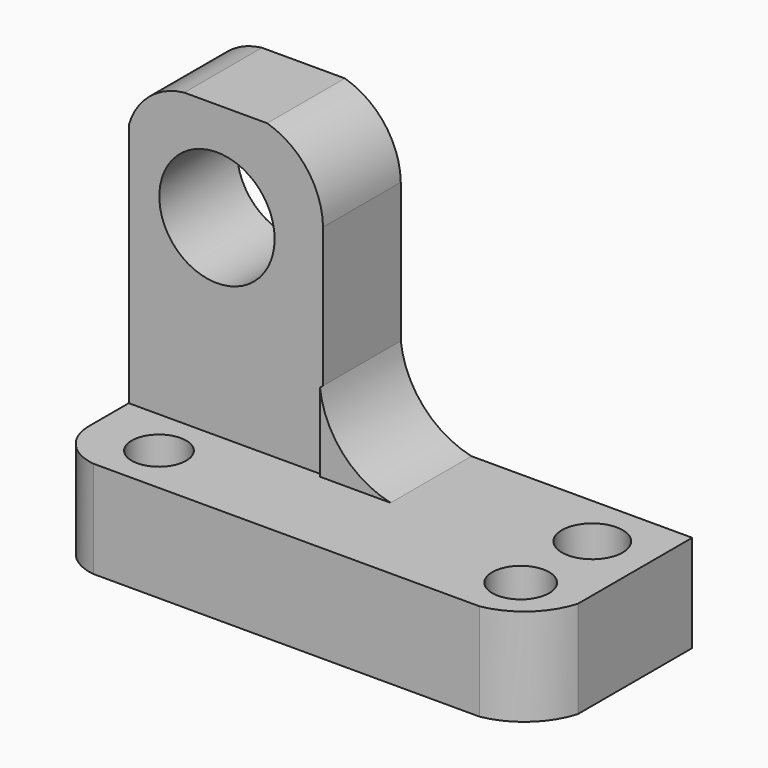
from build123d import *

# Parameters (mm, degrees)
F1_DEPTH  = 25.4
F3_DEPTH  = 25.4
F5_DEPTH  = 12.7
F6_R      = 7.5359717886
F7_DEPTH  = 25.4
F9_DEPTH  = 25.4
F11_DEPTH = 13.208
F12_R     = 3.5651940515
F12_R_2   = 3.719082418
F13_DEPTH = 25.4
F14_R     = 3.972943494
F15_DEPTH = 25.4


# Not quite as in the source:
# - a feature names something its author has since deleted; it is built from what else it names


with BuildPart() as f1:
    # F0 (on Front) → F1 (new body)
    with BuildSketch(Plane.XZ):
        Polygon((-56.0294090864, 50.8), (-56.0294090864, 0), (7.4705909136, 0), (7.4705909136, 12.7), (-30.6294090864, 12.7), (-30.6294090864, 50.8), align=None)
    extrude(amount=F1_DEPTH)

    # F2 (on face) → F3 (cut)
    with BuildSketch(Plane.XZ.offset(25.4)):
        with BuildLine():
            ThreePointArc((-56.0294090864, 44.6911064088), (-53.33876103, 48.8568702153), (-48.7761497498, 50.8))
            Line((-48.7761497498, 50.8), (-56.0294090864, 50.8))
            Line((-56.0294090864, 50.8), (-56.0294090864, 44.6911064088))
        make_face()
        with BuildLine():
            Line((-30.6294090864, 50.8), (-37.9370041192, 50.8))
            ThreePointArc((-37.9370041192, 50.8), (-32.7129588614, 47.2060747706), (-30.6294090864, 41.2172712386))
            Line((-30.6294090864, 41.2172712386), (-30.6294090864, 50.8))
        make_face()
    extrude(amount=-F3_DEPTH, mode=Mode.SUBTRACT)

    # F4 (on face) → F5 (cut)
    with BuildSketch(Plane.XZ.offset(25.4)):
        with BuildLine():
            Line((-56.0294090864, 12.7), (-30.6294090864, 12.7))
            Line((-30.6294090864, 12.7), (-30.6294090864, 41.2172712386))
            ThreePointArc((-30.6294090864, 41.2172712386), (-32.7129588614, 47.2060747706), (-37.9370041192, 50.8))
            Line((-37.9370041192, 50.8), (-48.7761497498, 50.8))
            ThreePointArc((-48.7761497498, 50.8), (-53.33876103, 48.8568702153), (-56.0294090864, 44.6911064088))
            Line((-56.0294090864, 44.6911064088), (-56.0294090864, 12.7))
        make_face()
    extrude(amount=-F5_DEPTH, mode=Mode.SUBTRACT)

    # F6 (on face) → F7 (cut)
    with BuildSketch(Plane.XZ.offset(12.7)):
        with Locations((-44.4975420833, 37.7943851054)):
            Circle(F6_R)
    extrude(amount=-F7_DEPTH, mode=Mode.SUBTRACT)

    # F8 (on face) → F9 (cut)
    with BuildSketch(Plane.XY.offset(12.7)):
        with BuildLine():
            Line((-56.0294090864, -25.4), (-50.4875965416, -25.4))
            ThreePointArc((-50.4875965416, -25.4), (-54.4030732732, -23.3868988254), (-56.0294090864, -19.2956195392))
            Line((-56.0294090864, -19.2956195392), (-56.0294090864, -25.4))
        make_face()
        with BuildLine():
            ThreePointArc((7.4705909136, -18.6832621694), (4.6896834238, -23.1031347869), (0, -25.4))
            Line((0, -25.4), (7.4705909136, -25.4))
            Line((7.4705909136, -25.4), (7.4705909136, -18.6832621694))
        make_face()
    extrude(amount=-F9_DEPTH, mode=Mode.SUBTRACT)

    # F10 (on face) → F11 (join)
    with BuildSketch(Plane(origin=(0, 0, 0), x_dir=(-1, 0, 0), z_dir=(0, 1, 0))):
        with BuildLine():
            ThreePointArc((30.6294090864, 22.9618716985), (27.6481288956, 16.3576173964), (21.3930476457, 12.7))
            Line((21.3930476457, 12.7), (30.6294090864, 12.7))
            Line((30.6294090864, 12.7), (30.6294090864, 22.9618716985))
        make_face()
    extrude(amount=-F11_DEPTH)

    # F12 (on face) → F13 (cut)
    with BuildSketch(Plane.XY.offset(12.7)):
        with Locations((-47.0647066832, -18.9685039222)):
            Circle(F12_R)
        with Locations((0, -18.6832621694)):
            Circle(F12_R_2)
    extrude(amount=-F13_DEPTH, mode=Mode.SUBTRACT)

    # F14 (on face) → F15 (cut)
    with BuildSketch(Plane.XY.offset(12.7)):
        with Locations((0, -6.9883959368)):
            Circle(F14_R)
    extrude(amount=-F15_DEPTH, mode=Mode.SUBTRACT)


solid = f1.part
